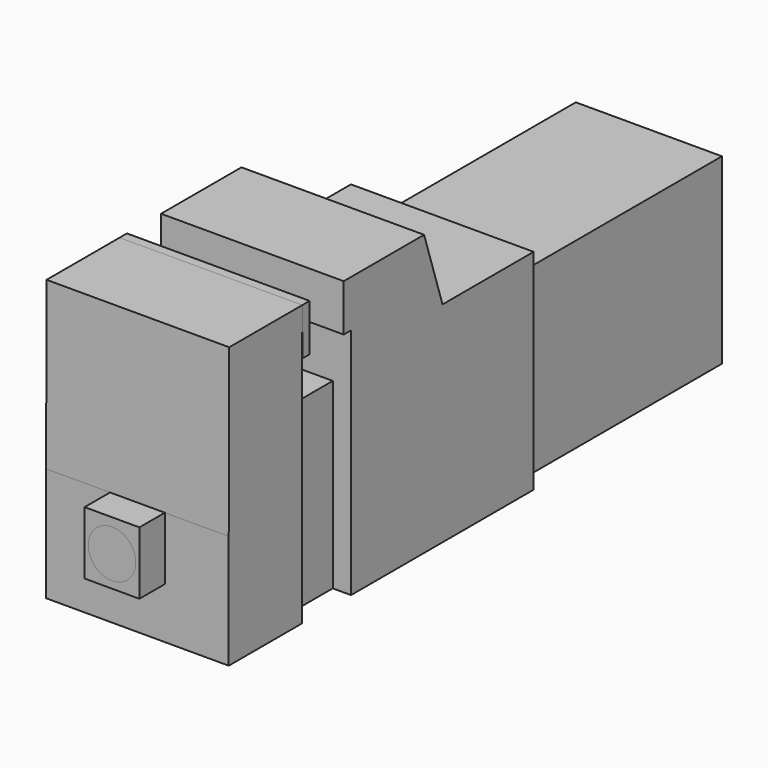
from build123d import *

# Parameters (mm, degrees)
F0_W        = 124.9519532199
F0_H        = 100
F1_DEPTH    = 50
F0_W_2      = 141.3618674554
F2_DEPTH    = 40
F0_W_3      = 5
F0_H_2      = 25.7300529629
F3_DEPTH    = 50
F4_DEPTH    = 50
F0_W_4      = 17.3817112001
F0_H_3      = 34.4321173714
F5_DEPTH    = 15
F6_T        = 2.5
F6_T3_DEPTH = 105
F6_T5_DEPTH = 105
F6_T7_DEPTH = 85
F7_R        = 13
F8_DEPTH    = 330


# Not quite as in the source:
# - a shell that OpenCascade refuses in one call is made with other operations: the cavity is built on its own and cut out


with BuildPart() as f1:
    # F0 (on Right) → F1 (new body, symmetric)
    with BuildSketch(Plane.YZ):
        Polygon((-82.4616801739, -53.3395072201), (42.490273046, -53.3395072201), (42.490273046, -38.6770403606), (0, -38.6770403606), (-19.8455593103, -38.6770403606), (-32.4616801739, 0), (-77.4616801739, 0), (-82.4616801739, 0), (-82.4616801739, -25.7300529629), align=None)
        with Locations((-19.9857035639, -103.3395072201)):
            Rectangle(F0_W, F0_H)
    extrude(amount=F1_DEPTH, both=True)

    # F0 (on Right) → F2 (join, symmetric)
    with BuildSketch(Plane.YZ):
        with Locations((113.1712067737, -103.3395072201)):
            Rectangle(F0_W_2, F0_H)
        Polygon((-116.1451248146, -153.3395072201), (-82.4616801739, -153.3395072201), (-82.4616801739, -53.3395072201), (-115.929015638, -53.3395072201), align=None)
    extrude(amount=F2_DEPTH, both=True)

    # F0 (on Right) → F3, piece 2 (join, symmetric)
    with BuildSketch(Plane.YZ):
        Polygon((-82.4616801739, -53.3395072201), (42.490273046, -53.3395072201), (42.490273046, -38.6770403606), (0, -38.6770403606), (-19.8455593103, -38.6770403606), (-32.4616801739, 0), (-77.4616801739, 0), (-82.4616801739, 0), (-82.4616801739, -25.7300529629), align=None)
    extrude(amount=F3_DEPTH, both=True)

    # F0 (on Right) → F4 (join, symmetric)
    with BuildSketch(Plane.YZ):
        with Locations((-84.9616801739, -12.8650264814)):
            Rectangle(F0_W_3, F0_H_2)
    extrude(amount=F4_DEPTH, both=True)

    # F6: shell of thickness 2.5, made by hand


with BuildPart() as f1b:
    # F0 (on Right) → F1, piece 2 (new body, symmetric)
    with BuildSketch(Plane.YZ):
        Polygon((-166.1478594986, -153.3395072201), (-116.1451248146, -153.3395072201), (-116.1451248146, -53.3395072201), (-115.929015638, -53.3395072201), (-115.8137440681, 0), (-165.8137440681, 0), (-166.1478594986, -90.9727620794), (-166.1478594986, -125.4048794508), align=None)
    extrude(amount=F1_DEPTH, both=True)

    # F0 (on Right) → F5 (join, symmetric)
    with BuildSketch(Plane.YZ):
        with Locations((-174.8387150987, -108.1888207651)):
            Rectangle(F0_W_4, F0_H_3)
    extrude(amount=F5_DEPTH, both=True)


with BuildPart() as f3:
    # F0 (on Right) → F3 (new body, symmetric)
    with BuildSketch(Plane.YZ):
        with Locations((-113.3137440681, -12.8650264814)):
            Rectangle(F0_W_3, F0_H_2)
    extrude(amount=F3_DEPTH, both=True)


with BuildPart() as f6_core1:
    # F6_t2: copy of F1
    add(f1.part)

    # the walls: a layer under each face that stays
    f6_faces = [f6_core1.faces().sort_by_distance(p)[0] for p in [
        (-33.3333333333, -82.4616801739, -46.9982953391),
        (-50, -22.4857035639, -76.66975361),
        (0, -87.4616801739, -12.8650264814),
        (0, -59.9616801739, 0),
        (0, -26.1536197421, -19.3385201803),
        (0, 11.3223568678, -38.6770403606),
        (-42.8571428571, 42.490273046, -145.1493310158),
        (40, 113.1712067737, -103.3395072201),
        (0, 183.8521405014, -103.3395072201),
        (-40, 113.1712067737, -103.3395072201),
        (0, 113.1712067737, -53.3395072201),
        (-40, -99.3034024943, -103.3395072201),
        (0, -116.0370702263, -103.3395072201),
        (0, -99.1953479059, -53.3395072201),
        (40, -99.3034024943, -103.3395072201),
        (50, -22.4857035639, -76.66975361),
        (0, -84.9616801739, -25.7300529629),
    ]]
    thicken(f6_faces, amount=-F6_T, mode=Mode.SUBTRACT)

    # F6_s4 → F6_t3 (cut)
    with BuildSketch(Plane.YZ.offset(-52.5)):
        Polygon((-82.4866801739, -25.7550529629), (-79.9616801739, -25.7300529629), (-79.9616801739, -23.2300529629), (-82.4616801739, -23.2300529629), align=None)
        Polygon((-19.8217917967, -38.6442876003), (-22.222310679, -39.4523163965), (-21.6597204242, -41.1770403606), (-19.8455593103, -41.1770403606), align=None)
    extrude(amount=F6_T3_DEPTH, mode=Mode.SUBTRACT)

    # F6_s6 → F6_t5 (cut)
    with BuildSketch(Plane.XY.offset(-155.8395072201)):
        Polygon((40.025, -82.4866801739), (40, -79.9616801739), (37.5, -79.9616801739), (37.5, -82.4616801739), align=None)
        Polygon((-40.025, -82.4866801739), (-40, -79.9616801739), (-37.5, -79.9616801739), (-37.5, -82.4616801739), align=None)
        Polygon((-40.025, 42.515273046), (-40, 39.990273046), (-37.5, 39.990273046), (-37.5, 42.490273046), align=None)
        Polygon((40.025, 42.515273046), (40, 39.990273046), (37.5, 39.990273046), (37.5, 42.490273046), align=None)
    extrude(amount=F6_T5_DEPTH, mode=Mode.SUBTRACT)

    # F6_s8 → F6_t7 (cut)
    with BuildSketch(Plane.YZ.offset(-42.5)):
        Polygon((-82.4866801739, -53.3145072201), (-79.9616801739, -53.3395072201), (-79.9616801739, -55.8395072201), (-82.4616801739, -55.8395072201), align=None)
        Polygon((42.515273046, -53.3145072201), (39.990273046, -53.3395072201), (39.990273046, -55.8395072201), (42.490273046, -55.8395072201), align=None)
    extrude(amount=F6_T7_DEPTH, mode=Mode.SUBTRACT)


with BuildPart() as f1_1:
    add(f1.part)

    # what is left inside the walls is the cavity
    f6_cavity = [f6_core1.part.solids().sort_by_distance(p)[0] for p in [
        (-15.833333, 33.853511, -153.314507),
    ]]
    add(f6_cavity, mode=Mode.SUBTRACT)


with BuildPart() as f8:
    # F7 (on face) → F8 (new body)
    with BuildSketch(Plane.XZ.offset(183.5295706987)):
        with Locations((0, -108.5942578374)):
            Circle(F7_R)
    extrude(amount=-F8_DEPTH)


solid = Compound([f1b.part, f3.part, f1_1.part, f8.part])
